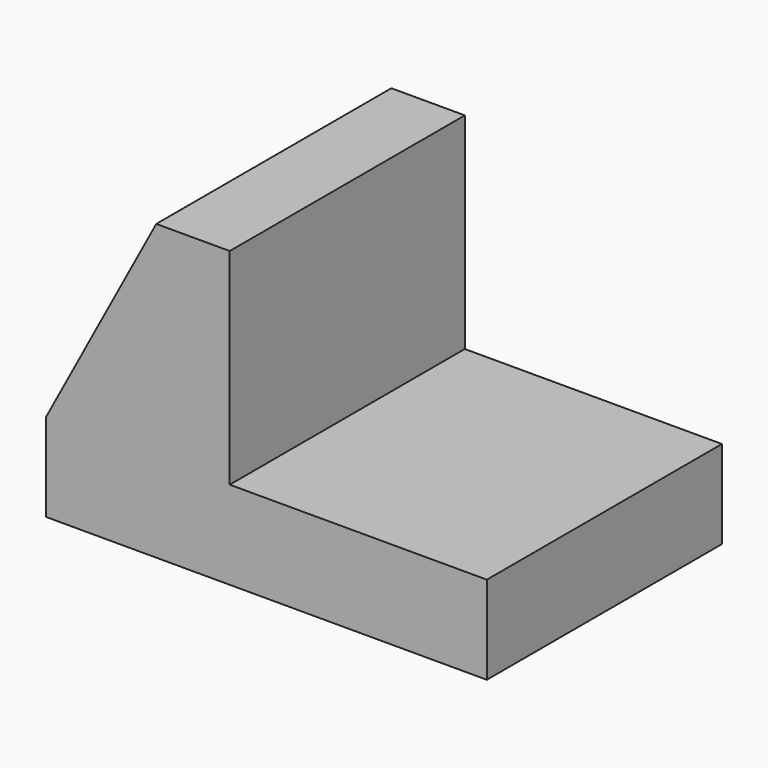
from build123d import *

# Parameters (mm, degrees)
F3_DEPTH = 12.7


# Not quite as in the source:
# - the program builds the solid bodies; features that only make, move or delete a surface that nothing else refers to are left out


with BuildPart() as f3:
    # F2 (on Front) → F3 (new body, symmetric)
    with BuildSketch(Plane.XZ):
        with BuildLine():
            Line((-22.225, 25.4), (-28.3980633142, 25.4))
            ThreePointArc((-28.3980633142, 25.4), (-28.6260297603, 25.1428005632), (-28.8516668522, 24.8835552092))
            Line((-28.8516668522, 24.8835552092), (-38.1, 7.62))
            Line((-38.1, 7.62), (-38.1, 0))
            Line((-38.1, 0), (0, 0))
            Line((0, 0), (0, 7.62))
            Line((0, 7.62), (-22.225, 7.62))
            Line((-22.225, 7.62), (-22.225, 25.4))
        make_face()
        with BuildLine():
            ThreePointArc((-28.8516668522, 24.8835552092), (-28.6260297603, 25.1428005632), (-28.3980633142, 25.4))
            Line((-28.3980633142, 25.4), (-28.575, 25.4))
            Line((-28.575, 25.4), (-28.8516668522, 24.8835552092))
        make_face()
    extrude(amount=F3_DEPTH, both=True)


solid = f3.part
